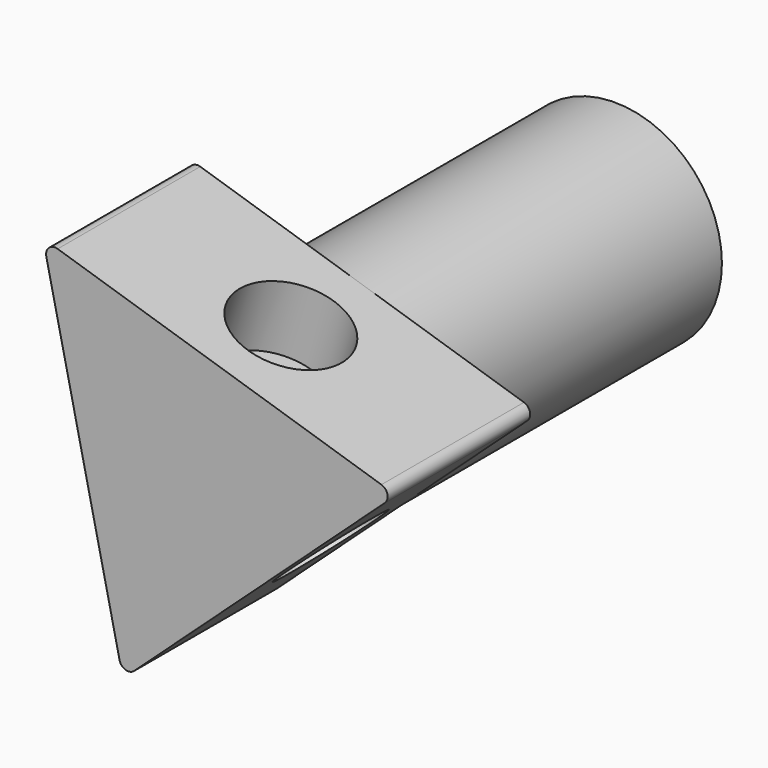
from build123d import *

# Parameters (mm, degrees)
F0_R            = 3
F1_DEPTH        = 10
F3_DEPTH        = 5
F5_R            = 1.5
F6_DEPTH        = 2
F6_COPIES_COUNT = 3
F7_R            = 0.25


# Not quite as in the source:
# - a pattern or mirror of a feature is missing from the dataset's text; its kind, count and spacing are read off the source's solid


with BuildPart() as f1:
    # F0 (on Front) → F1 (new body)
    with BuildSketch(Plane.XZ):
        Circle(F0_R)
    extrude(amount=F1_DEPTH)

    # F2 (on face) → F3 (join)
    with BuildSketch(Plane.XZ.offset(10)):
        Polygon((5.858499572, 1.2953697407), (-4.0510728887, 4.4259245871), (-1.8074266833, -5.7212943277), align=None)
    extrude(amount=F3_DEPTH)

    # F5 (on face) → F6 (cut)
    with BuildSketch(Plane(origin=(2.0255364444, 0, -2.2129622935), x_dir=(0.7376540978, 0, 0.6751788148), z_dir=(0.6751788148, 0, -0.7376540978))):
        with Locations((0, 12.5)):
            Circle(F5_R)
    f6 = extrude(amount=-F6_DEPTH, mode=Mode.SUBTRACT)

    # F6_copies: F6 ×3 about axis
    f6_copies_axis = Axis((0, 0, 0), (0, 1, 0))
    for i in range(1, F6_COPIES_COUNT):
        add(f6.rotate(f6_copies_axis, i * 360 / F6_COPIES_COUNT), mode=Mode.SUBTRACT)

    # F7
    f7_edges = [f1.edges().sort_by_distance(p)[0] for p in [
        (5.8585, -12.5, 1.29537),
        (-4.051073, -12.5, 4.425925),
        (-1.807427, -12.5, -5.721294),
    ]]
    fillet(f7_edges, radius=F7_R)


solid = f1.part
